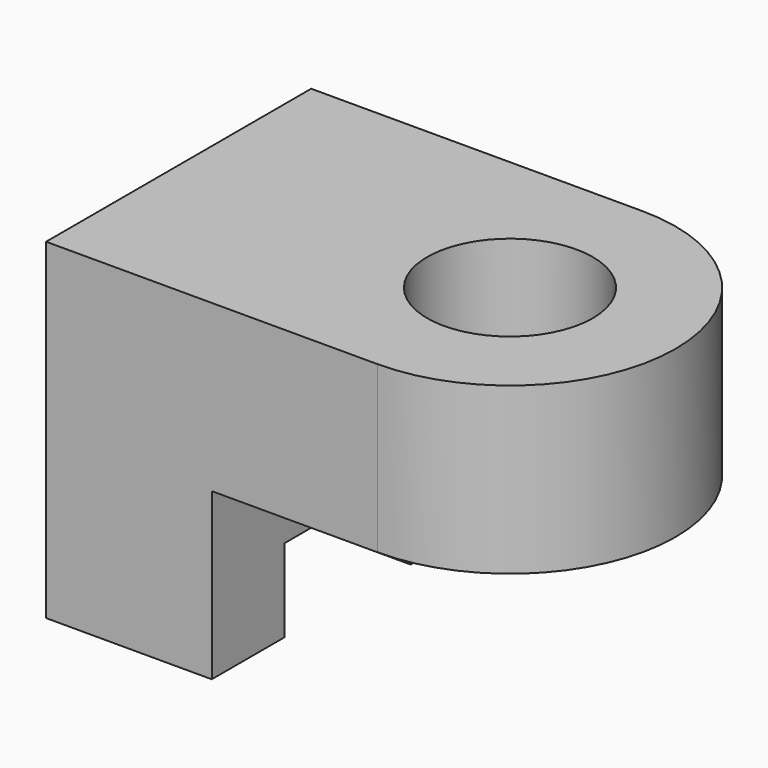
from build123d import *

# Parameters (mm, degrees)
F1_DEPTH = 25.4
F2_R     = 6.35
F3_DEPTH = 12.7
F4_DEPTH = 25.4
F5_W     = 12.7
F5_H     = 25.4
F6_DEPTH = 12.7
F7_W     = 12.7
F7_H     = 12.0984496011
F8_DEPTH = 6.35


# Not quite as in the source:
# - a feature names something its author has since deleted; it is built from what else it names


with BuildPart() as f1:
    # F0 (on Front) → F1 (new body)
    with BuildSketch(Plane.XZ):
        Polygon((0, 12.7), (0, 0), (0, -25.4), (12.7, -25.4), (12.7, 0), (58.456916362, 0), (58.456916362, 12.7), align=None)
    extrude(amount=F1_DEPTH)

    # F2 (on face) → F3 (cut, through all)
    with BuildSketch(Plane(origin=(0, 0, 0), x_dir=(1, 0, 0), z_dir=(0, 0, -1))):
        with Locations((25.4, 12.7)):
            Circle(F2_R)
        with BuildLine():
            ThreePointArc((25.4, 25.4), (38.1, 12.7), (25.4, 0))
            Line((25.4, 0), (58.456916362, 0))
            Line((58.456916362, 0), (58.456916362, 25.4))
            Line((58.456916362, 25.4), (25.4, 25.4))
        make_face()
    extrude(amount=-F3_DEPTH, mode=Mode.SUBTRACT)

    # F4 (cut): a face of the model
    f4_faces = [f1.faces().sort_by_distance(p)[0] for p in [
        (12.7, -12.7, -12.7),
    ]]
    extrude(f4_faces, amount=-F4_DEPTH, mode=Mode.SUBTRACT)

    # F5 (on face) → F6 (join)
    with BuildSketch(Plane(origin=(0, 0, 0), x_dir=(1, 0, 0), z_dir=(0, 0, -1))):
        with Locations((6.35, 12.7)):
            Rectangle(F5_W, F5_H)
    extrude(amount=F6_DEPTH)

    # F7 (on face) → F8 (cut)
    with BuildSketch(Plane(origin=(0, 0, -12.7), x_dir=(1, 0, 0), z_dir=(0, 0, -1))):
        with Locations((6.35, 12.3992248707)):
            Rectangle(F7_W, F7_H)
    extrude(amount=-F8_DEPTH, mode=Mode.SUBTRACT)


solid = f1.part
